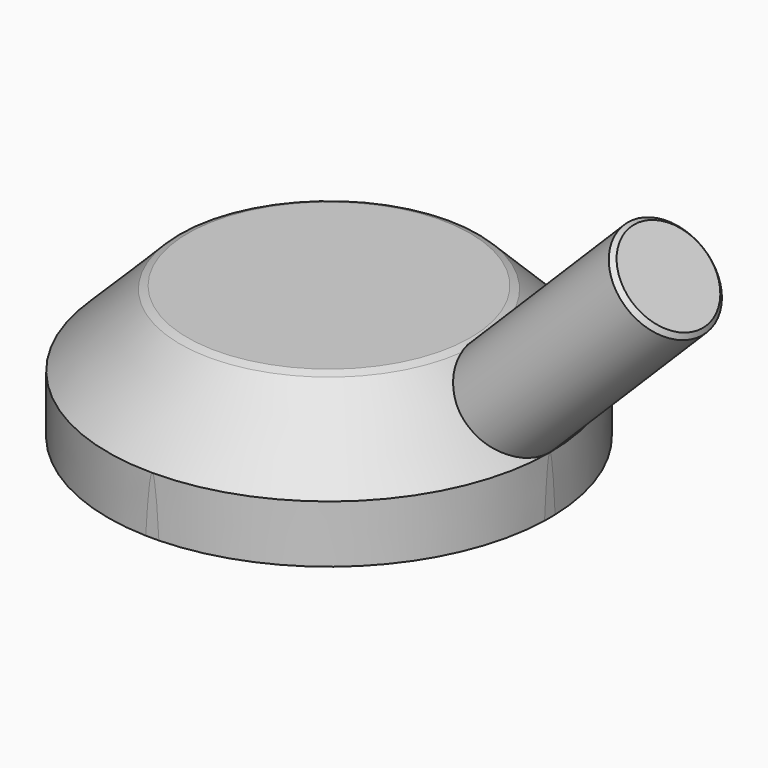
from build123d import *

# Parameters (mm, degrees)
F0_W          = 50
F0_H          = 50
F1_DEPTH      = 15
F2_SIZE       = 8.5
F3_R          = 6
F6_DEPTH      = 25
F6_DEPTH_BACK = 5
F7_SIZE       = 0.5
F7_2_SIZE     = 0.5


# Not quite as in the source:
# - a feature names something its author has since deleted; it is built from what else it names


with BuildPart() as f1:
    # F0 (on Top) → F1 (new body)
    with BuildSketch(Plane.XY):
        Rectangle(F0_W, F0_H)
    extrude(amount=-F1_DEPTH)

    # F2
    f2_edges = [f1.edges().sort_by_distance(p)[0] for p in [
        (25, 0, 0),
    ]]
    chamfer(f2_edges, length=F2_SIZE)

    # F4 (on Front) → F5 (revolve, cut)
    with BuildSketch(Plane.XZ):
        Polygon((16.5, 0), (25, -8.5), (25.0111613423, -15), (57.6415769756, -15), (57.6415769756, 0), align=None)
    revolve(axis=Axis((0, 0, -4.25), (0, 0, -1)), mode=Mode.SUBTRACT)

    # F7#2
    f7_2_edges = [f1.edges().sort_by_distance(p)[0] for p in [
        (-16.5, 0, 0),
    ]]
    chamfer(f7_2_edges, length=F7_2_SIZE)


with BuildPart() as f6:
    # F3 (on face) → F6 (new body, two sides)
    with BuildSketch(Plane(origin=(8.25, 0, 8.25), x_dir=(0, 1, 0), z_dir=(0.7071067812, 0, 0.7071067812))) as f6_sk:
        with Locations((0, -17.6776695297)):
            Circle(F3_R)
    extrude(amount=F6_DEPTH)
    extrude(f6_sk.sketch, amount=-F6_DEPTH_BACK)

    # F7
    f7_edges = [f6.edges().sort_by_distance(p)[0] for p in [
        (38.42767, -6, 13.42767),
    ]]
    chamfer(f7_edges, length=F7_SIZE)


solid = Compound([f1.part, f6.part])
